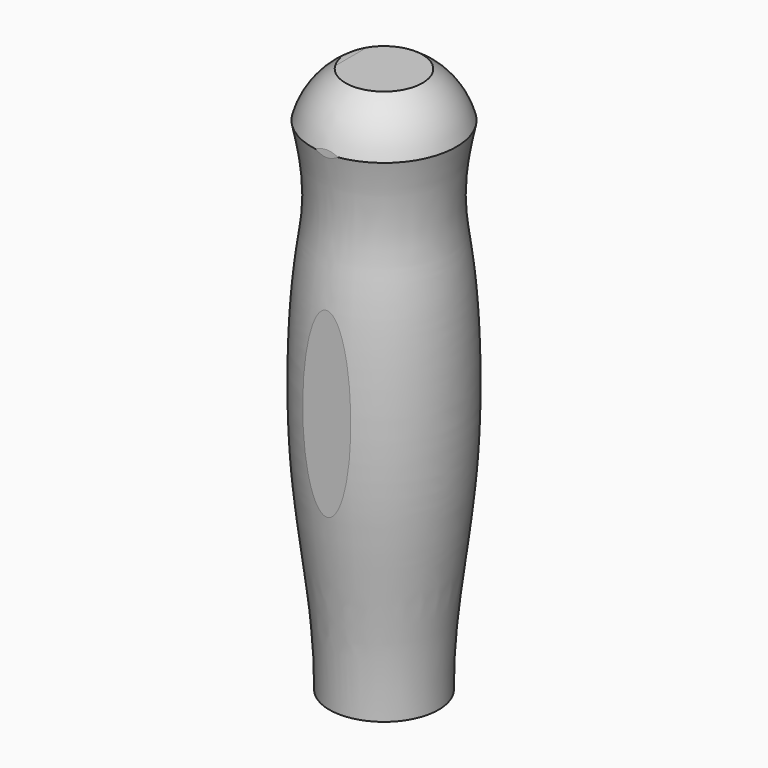
from build123d import *

# Parameters (mm, degrees)
F1_DEPTH    = 255
F3_T1_DEPTH = 120
F6_R        = 8
F7_DEPTH    = 1


# Not quite as in the source:
# - a fillet or chamfer that OpenCascade refuses, or shapes differently, is made with other operations: its cross-section is extruded or revolved along the edge and cut away or added
# - a feature of the source that left no trace in its solid (it failed there, or was rolled back) is left out


with BuildPart() as f1:
    # F0 (on Top) → F1 (new body)
    with BuildSketch(Plane.XY):
        with BuildLine():
            Line((25, 32.5), (-20, 32.5))
            ThreePointArc((-20, 32.5), (-27.0710678119, 29.5710678119), (-30, 22.5))
            Line((-30, 22.5), (-30, -22.5))
            ThreePointArc((-30, -22.5), (-27.0710678119, -29.5710678119), (-20, -32.5))
            Line((-20, -32.5), (25, -32.5))
            ThreePointArc((25, -32.5), (32.0710678119, -29.5710678119), (35, -22.5))
            Line((35, -22.5), (35, 22.5))
            ThreePointArc((35, 22.5), (32.0710678119, 29.5710678119), (25, 32.5))
        make_face()
    extrude(amount=F1_DEPTH)

    # F3: fillet of radius 15 on 1 edges, made by hand

    # F3_s2 → F3_t1 (cut)
    with BuildSketch(Plane.XZ.offset(-60)):
        with BuildLine():
            ThreePointArc((-30, 240), (-25.6066017178, 250.6066017178), (-15, 255))
            Line((-15, 255), (-30, 255))
            Line((-30, 255), (-30, 240))
        make_face()
    extrude(amount=F3_T1_DEPTH, mode=Mode.SUBTRACT)

    # F4 (on Right) → F5 (revolve, cut)
    with BuildSketch(Plane.YZ):
        with BuildLine():
            Line((-81.634151806, 0), (-25, 0))
            add(Edge.make_bspline(
                [(-25, 0), (-23.6501835563, 32.3706567612), (-36.5171185658, 88.4711609326), (-33.6122660538, 175.7126997283), (-27.0812273729, 203.3899516553), (-32.6822734448, 236.8273684293), (-37.4866381261, 250.6565702698), (-43.8172206407, 257)],
                knots=[0, 0, 0, 0, 0.2659510877, 0.5166221716, 0.6640954741, 0.8227476521, 0.9335873904, 0.9335873904, 0.9335873904, 0.9335873904], degree=3))
            Line((-43.8172206407, 257), (-81.634151806, 257))
            Line((-81.634151806, 257), (-81.634151806, 0))
        make_face()
    revolve(axis=Axis((0, 0, 144.3710991352), (0, 0, 1)), mode=Mode.SUBTRACT)

    # F6 (on face) → F7 (cut)
    with BuildSketch(Plane(origin=(0, 0, 0), x_dir=(1, 0, 0), z_dir=(0, 0, -1))):
        Circle(F6_R)
    extrude(amount=-F7_DEPTH, mode=Mode.SUBTRACT)

    # F8 (on Right) → F9 (revolve, cut)
    with BuildSketch(Plane.YZ):
        with BuildLine():
            ThreePointArc((-34, 225.8460643248), (-24.0416305603, 249.8876948852), (0, 259.8460643248))
            Line((0, 259.8460643248), (0, 291.8460643248))
            Line((0, 291.8460643248), (-96, 291.8460643248))
            Line((-96, 291.8460643248), (-96, 225.8460643248))
            Line((-96, 225.8460643248), (-34, 225.8460643248))
        make_face()
    revolve(axis=Axis((0, 0, 221.1364358664), (0, 0, -1)), mode=Mode.SUBTRACT)

    # F10 (on Right) → F12 (revolve, cut)
    with BuildSketch(Plane.YZ):
        with BuildLine():
            ThreePointArc((0, 0), (-35.3553390593, 14.6446609407), (-50, 50))
            Line((-50, 50), (-50, -21.7864606529))
            Line((-50, -21.7864606529), (0, -21.7864606529))
            Line((0, -21.7864606529), (0, 0))
        make_face()
    revolve(axis=Axis((0, 0, 34.5914699137), (0, 0, 1)), mode=Mode.SUBTRACT)


solid = f1.part
